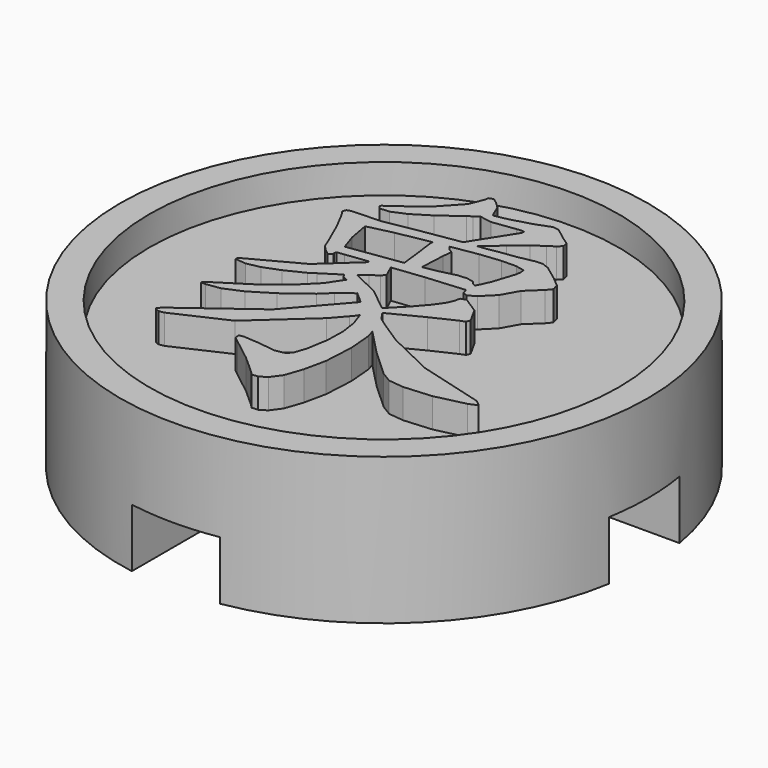
from build123d import *

# Parameters (mm, degrees)
F0_R     = 9
F1_DEPTH = 4
F3_W     = 3
F3_H     = 3
F4_DEPTH = 2
F2_R     = 9
F2_R_2   = 8
F5_DEPTH = 1
F7_DEPTH = 1


# Not quite as in the source:
# - a feature names something its author has since deleted; it is built from what else it names


with BuildPart() as f1:
    # F0 (on Top) → F1 (new body)
    with BuildSketch(Plane.XY):
        with Locations((-31.3306450844, 19.7580661625)):
            Circle(F0_R)
    extrude(amount=F1_DEPTH)

    # F3 (on face) → F4 (cut)
    with BuildSketch(Plane(origin=(0, 0, 0), x_dir=(1, 0, 0), z_dir=(0, 0, -1))):
        with BuildLine():
            ThreePointArc((-32.8306450844, -28.6321858371), (-32.0832814269, -28.7265408676), (-31.3306450844, -28.7580661625))
            ThreePointArc((-31.3306450844, -28.7580661625), (-30.5780087419, -28.7265408676), (-29.8306450844, -28.6321858371))
            Line((-29.8306450844, -28.6321858371), (-29.8306450844, -21.2580661625))
            Line((-29.8306450844, -21.2580661625), (-32.8306450844, -21.2580661625))
            Line((-32.8306450844, -21.2580661625), (-32.8306450844, -28.6321858371))
        make_face()
        with BuildLine():
            ThreePointArc((-40.204764759, -18.2580661625), (-40.2991197895, -19.0054298199), (-40.3306450844, -19.7580661625))
            ThreePointArc((-40.3306450844, -19.7580661625), (-40.2991197895, -20.510702505), (-40.204764759, -21.2580661625))
            Line((-40.204764759, -21.2580661625), (-32.8306450844, -21.2580661625))
            Line((-32.8306450844, -21.2580661625), (-32.8306450844, -18.2580661625))
            Line((-32.8306450844, -18.2580661625), (-40.204764759, -18.2580661625))
        make_face()
        with Locations((-31.3306450844, -19.7580661625)):
            Rectangle(F3_W, F3_H)
        with BuildLine():
            Line((-29.8306450844, -18.2580661625), (-29.8306450844, -21.2580661625))
            Line((-29.8306450844, -21.2580661625), (-22.4565254097, -21.2580661625))
            ThreePointArc((-22.4565254097, -21.2580661625), (-22.3621703793, -20.510702505), (-22.3306450844, -19.7580661625))
            ThreePointArc((-22.3306450844, -19.7580661625), (-22.3621703793, -19.0054298199), (-22.4565254097, -18.2580661625))
            Line((-22.4565254097, -18.2580661625), (-29.8306450844, -18.2580661625))
        make_face()
        with BuildLine():
            Line((-32.8306450844, -10.8839464878), (-32.8306450844, -18.2580661625))
            Line((-32.8306450844, -18.2580661625), (-29.8306450844, -18.2580661625))
            Line((-29.8306450844, -18.2580661625), (-29.8306450844, -10.8839464878))
            ThreePointArc((-29.8306450844, -10.8839464878), (-30.5780087419, -10.7895914574), (-31.3306450844, -10.7580661625))
            ThreePointArc((-31.3306450844, -10.7580661625), (-32.0832814269, -10.7895914574), (-32.8306450844, -10.8839464878))
        make_face()
    extrude(amount=-F4_DEPTH, mode=Mode.SUBTRACT)

    # F2 (on face) → F5 (join)
    with BuildSketch(Plane.XY.offset(4)):
        with Locations((-31.3306450844, 19.7580661625)):
            Circle(F2_R)
        with Locations((-31.3306450844, 19.7580661625)):
            Circle(F2_R_2, mode=Mode.SUBTRACT)
    extrude(amount=F5_DEPTH)

    # F6 (on face) → F7 (join)
    with BuildSketch(Plane.XY.offset(4)):
        Polygon((-30.381766284, 17.9040319534), (-30.4619589735, 18.1746830381), (-29.6149013378, 17.2983889264), (-28.7044060656, 16.4638793947), (-28.3493614045, 16.2516952002), (-27.8356165687, 16.1932222482), (-26.8858402754, 16.2684078198), (-25.8809008198, 16.5039787704), (-25.606903574, 16.6209307364), (-25.657884035, 16.6852352227), (-25.7906999566, 16.7879902517), (-28.0636647188, 17.4136738737), (-29.6733985374, 18.1880434347), (-29.9707886011, 18.3818358672), (-30.4444279992, 18.6900827686), (-30.7326343057, 18.8997573424), (-30.9264206763, 19.1837748856), (-29.8279160107, 19.7442932334), (-29.0385372201, 20.1160323285), (-28.8706229788, 20.1795245221), (-28.8180058086, 20.309824761), (-29.1053392034, 20.827752298), (-29.6466656203, 21.1786142578), (-29.8187625629, 21.1192683942), (-29.8671970318, 20.9313499292), (-29.9532333793, 20.7191233015), (-30.1829485481, 20.3908721764), (-30.5647140025, 19.9489728131), (-31.1068708977, 19.3909519623), (-31.9029480724, 20.0350030988), (-32.8176684792, 20.4668882264), (-32.5720590455, 20.6773569072), (-32.3131074007, 20.827752298), (-32.2095218933, 20.9714189954), (-32.3899660529, 21.3724127522), (-31.3298937444, 21.4943778978), (-30.0242544353, 21.6062803128), (-30.0108879768, 21.5929441637), (-29.9599257014, 21.4316979969), (-29.8037290857, 21.3724127522), (-29.554767429, 21.5169281136), (-29.1421348513, 21.9304093554), (-28.835524659, 22.4792525109), (-28.3669408738, 22.9261347444), (-28.2232135575, 23.0990803511), (-28.2900761597, 23.3237944639), (-28.6233586502, 23.6044597842), (-29.1187359714, 23.9719919303), (-29.3676370092, 24.0622534124), (-29.5965338234, 24.0488566444), (-30.1228146393, 23.943622304), (-30.6691421121, 23.868454918), (-31.0433787041, 23.8032896439), (-31.3674895611, 23.7648572868), (-30.767702316, 24.2769047945), (-30.2840365584, 24.6678964394), (-29.9256942314, 24.9351649917), (-29.7001314545, 25.0713149505), (-29.567315533, 25.2049795361), (-29.6099305913, 25.382107844), (-29.869682405, 25.5625095704), (-30.244773723, 25.8499035841), (-30.4644625324, 25.8883359412), (-30.6424091949, 25.823170667), (-30.9823840075, 25.6936887828), (-31.6782339596, 25.4990416243), (-31.9380403303, 25.4422417528), (-32.1426956624, 25.4088407612), (-32.2128559306, 25.5591755331), (-32.3365062805, 25.8499035841), (-32.5503574937, 26.049521489), (-32.7007104513, 26.1606358588), (-32.848565912, 26.1188694645), (-32.8811364253, 25.9668373644), (-33.0732800248, 25.5023756616), (-33.7098083608, 24.81404851), (-34.6687987208, 24.0755895615), (-34.8024511826, 24.0012708396), (-34.835864298, 23.9586557812), (-34.7590117077, 23.8417220009), (-34.4273780502, 23.8634235527), (-33.9595823101, 24.0622534124), (-33.366493449, 24.4273001853), (-32.6606171375, 24.9443790583), (-32.5169322545, 25.0396112869), (-32.3498727391, 25.1515137018), (-31.9397073489, 25.0830143904), (-31.1603306701, 25.1883093497), (-31.0091169246, 25.2058282001), (-30.899693821, 25.2016454988), (-30.9080531618, 25.1197494194), (-30.9397871348, 25.0579788014), (-31.2822897539, 24.5199864218), (-31.7951859256, 23.7113914526), (-33.1417793362, 23.4941940784), (-34.2786860493, 23.2928788454), (-35.186714134, 23.2602658989), (-35.3345695947, 23.2301989445), (-35.3805126284, 23.2068000647), (-35.4214479382, 23.0781668445), (-35.3170264967, 22.9395315124), (-34.9920730375, 22.3146723069), (-34.6420658036, 21.5160794496), (-34.5393168365, 21.2495989425), (-34.3714086571, 21.0750166266), (-34.1842903611, 20.9238331906), (-34.0740246553, 21.0349475604), (-34.084887555, 21.0783506639), (-34.0606642586, 21.1518813407), (-33.8209227305, 21.1835850043), (-33.0381877669, 21.2821512701), (-33.0674242429, 21.2429308679), (-33.0615866467, 21.218683324), (-34.2026699993, 20.1753539446), (-35.9117981374, 19.2606335378), (-35.9251639897, 19.170408427), (-35.5559381526, 19.1353343548), (-35.0989986441, 19.2297300431), (-34.5568599345, 19.4368889341), (-33.9303458341, 19.7417957364), (-33.7156641426, 19.8813100419), (-33.1016799605, 20.273089732), (-33.0323501707, 20.1602962198), (-32.8677699667, 20.079273052), (-33.2228085659, 19.5480033039), (-33.8058650058, 18.9674201135), (-34.6261957862, 18.3367354356), (-35.6912667259, 17.656755501), (-35.8015318254, 17.5439922983), (-35.6411446279, 17.5398035351), (-35.163327378, 17.6091515105), (-34.555186854, 17.8689396955), (-33.8259237865, 18.316676655), (-32.9847279946, 18.9498891393), (-32.6422253755, 19.278164512), (-32.1694225176, 19.6382041671), (-32.1560560591, 19.6515706257), (-31.7684530084, 19.3140933101), (-33.3272306136, 17.5214360206), (-35.6912667259, 15.7655258838), (-35.8098857105, 15.6327039003), (-35.7547522514, 15.5850877861), (-35.6520038905, 15.5433213918), (-35.470734102, 15.5717213275), (-33.7106388391, 16.3786614018), (-31.8987774948, 18.0176316964), (-31.4894486449, 18.4837604179), (-31.3273901855, 18.6792380547), (-31.3340825076, 18.6834086322), (-31.3140237269, 18.7193374303), (-31.1544688264, 18.2440128279), (-31.0742761369, 17.695187858), (-31.0884791357, 17.0594778767), (-31.2104382195, 16.3235346108), (-31.3424236627, 15.9317609826), (-31.4844415271, 15.7655258838), (-31.8311147237, 15.7012032118), (-32.4400736023, 15.7788923423), (-32.951320941, 15.8131359362), (-33.1150464191, 15.7788923423), (-33.0841247388, 15.6285272609), (-32.9346022595, 15.5082351958), (-32.1527220218, 14.9017677523), (-31.6114016668, 14.4189379288), (-31.4259564513, 14.2393375838), (-31.2238046781, 14.2518681082), (-30.9823840075, 14.3997259936), (-30.7326343057, 14.7430554539), (-30.5287912663, 15.3369869172), (-30.3683998254, 16.0896428027), (-30.3132730345, 17.1037660155), align=None)
        Polygon((-32.2730140869, 21.8000788072), (-34.0974174733, 21.5394783294), (-34.2778495091, 22.0849268288), (-34.4081679336, 22.795864815), (-33.5636199188, 22.9946340559), (-32.4300654286, 23.2068000647), (-32.4292288883, 23.0865322471), (-32.3966401893, 22.82005174), (-32.3415073365, 22.3957197223), align=None, mode=Mode.SUBTRACT)
        Polygon((-30.0919172065, 21.9955746296), (-30.1645810336, 22.0974749327), (-30.4051651638, 22.1509407669), (-30.7326343057, 22.1242078498), (-31.2580603957, 21.9955746296), (-31.7550926118, 21.9036764383), (-31.7141566958, 22.7548864658), (-31.6782339596, 23.0664674046), (-31.8219188427, 23.1592142599), (-31.9121439534, 23.286998816), (-31.0333462828, 23.4323628415), (-30.3316647965, 23.5083788916), (-29.8262793015, 23.5158956302), (-29.5330658773, 23.4541250122), (-29.5071816242, 23.3287652104), (-29.5330658773, 23.1433321186), (-29.7761475046, 22.3957197223), (-29.9340293246, 22.0473431358), (-29.9841550596, 21.9538082353), align=None, mode=Mode.SUBTRACT)
    extrude(amount=F7_DEPTH)


solid = f1.part
